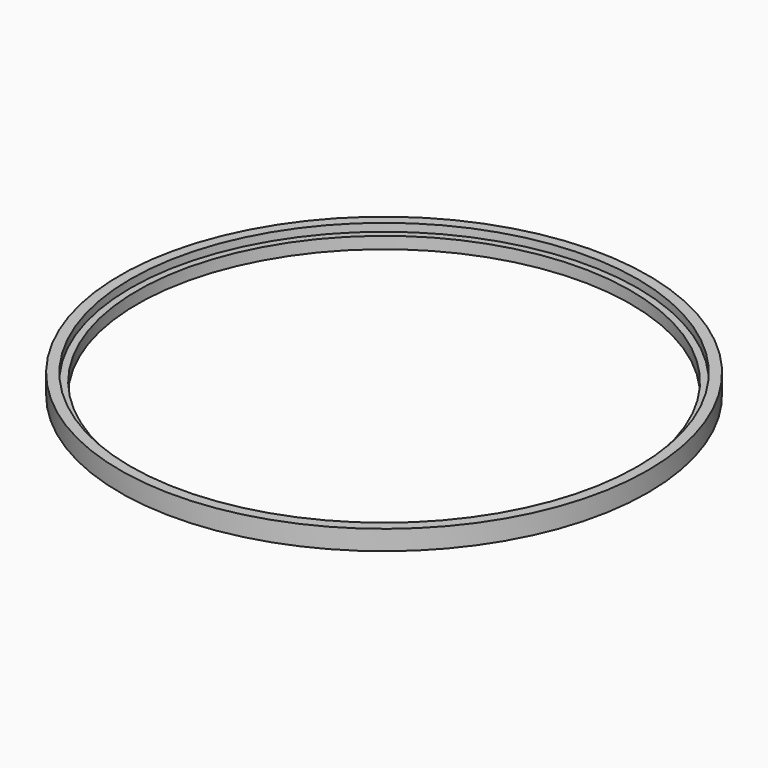
from build123d import *

# Parameters (mm, degrees)
F0_R     = 67
F0_R_2   = 64.375
F1_DEPTH = 5
F0_R_3   = 62.625
F2_DEPTH = 3
F0_R_4   = 58.875
F3_DEPTH = 2
F4_R     = 5.75
F5_DEPTH = 192


# Not quite as in the source:
# - an extrude ends at something that could not be found from the text; its depth is read off the source's solid


with BuildPart() as f1:
    # F0 (on Top) → F1 (new body)
    with BuildSketch(Plane.XY):
        Circle(F0_R)
        Circle(F0_R_2, mode=Mode.SUBTRACT)
    extrude(amount=F1_DEPTH)

    # F0 (on Top) → F2 (join)
    with BuildSketch(Plane.XY):
        Circle(F0_R_2)
        Circle(F0_R_3, mode=Mode.SUBTRACT)
    extrude(amount=F2_DEPTH)

    # F0 (on Top) → F3 (cut)
    with BuildSketch(Plane.XY):
        Circle(F0_R_3)
        Circle(F0_R_4, mode=Mode.SUBTRACT)
    extrude(amount=F3_DEPTH, mode=Mode.SUBTRACT)

    # F4 (on Top) → F5 (cut, through all)
    with BuildSketch(Plane.XY):
        with Locations((0, 46.25)):
            Circle(F4_R)
    extrude(amount=-F5_DEPTH, mode=Mode.SUBTRACT)


solid = f1.part
